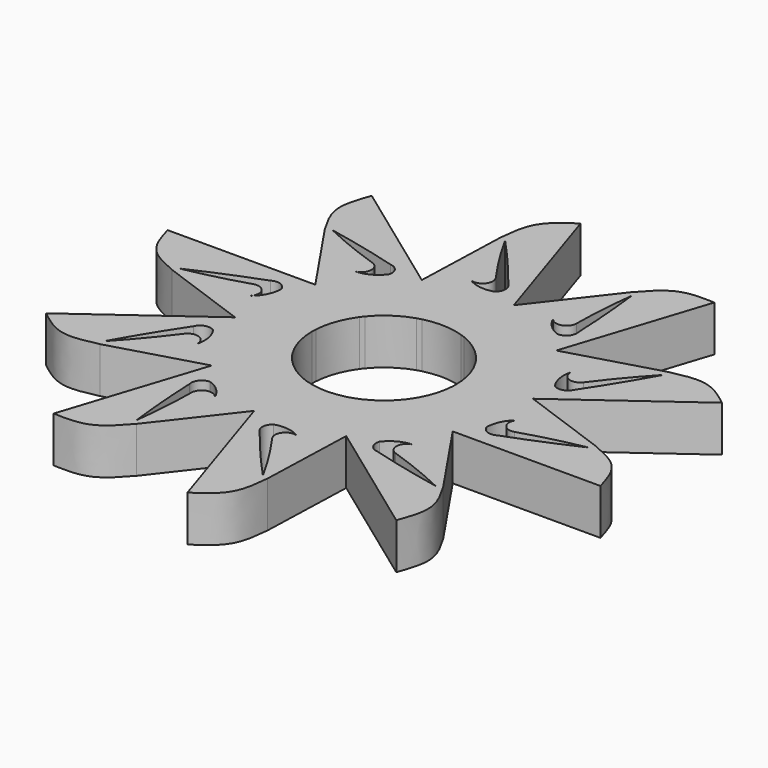
from build123d import *

# Parameters (mm, degrees)
F1_DEPTH      = 7
F3_DEPTH      = 80
F3_DEPTH_BACK = 25
F4_COUNT      = 10


# Not quite as in the source:
# - an extrude ends at something that could not be found from the text; its depth is read off the source's solid


with BuildPart() as f1:
    # F0 (on Top) → F1 (new body)
    with BuildSketch(Plane.XY):
        with BuildLine():
            ThreePointArc((9.2862347639, 5.8962567709), (10.5628732456, 3.0701317233), (11, 0))
            ThreePointArc((11, 0), (9.4389817008, -5.6485063912), (5.1989773724, -9.6938451752))
            Line((5.1989773724, -9.6938451752), (17.4936950276, -9.6938451752))
            ThreePointArc((17.4936950276, -9.6938451752), (19.3632887257, -5.0063010021), (20, 0))
            ThreePointArc((20, 0), (19.9371690623, 1.5840737934), (19.7490710217, 3.1581947026))
            Line((19.7490710217, 3.1581947026), (12.9913196682, 5.5989294212))
            ThreePointArc((12.9913196682, 5.5989294212), (12.1549883134, 5.8213640414), (11.2928291783, 5.8962567709))
            Line((11.2928291783, 5.8962567709), (9.2862347639, 5.8962567709))
        make_face()
        with BuildLine():
            ThreePointArc((5.1989773724, -9.6938451752), (-10.6404023576, 2.7895945347), (9.2862347639, 5.8962567709))
            Line((9.2862347639, 5.8962567709), (11.2928291783, 5.8962567709))
            ThreePointArc((11.2928291783, 5.8962567709), (12.1549883134, 5.8213640414), (12.9913196682, 5.5989294212))
            Line((12.9913196682, 5.5989294212), (19.7490710217, 3.1581947026))
            ThreePointArc((19.7490710217, 3.1581947026), (-19.6989755573, 3.4569295616), (17.4936950276, -9.6938451752))
            Line((17.4936950276, -9.6938451752), (5.1989773724, -9.6938451752))
        make_face()
        with BuildLine():
            ThreePointArc((20, 0), (19.3632887257, -5.0063010021), (17.4936950276, -9.6938451752))
            Line((17.4936950276, -9.6938451752), (40.8740527928, -9.6938451752))
            add(Edge.make_bspline(
                [(34.0516753495, -2.0075566135), (35.8141325987, -2.7740908853), (39.3168982789, -4.2975263847), (40.357193967, -7.9026709732), (40.8740527928, -9.6938451752)],
                knots=[0, 0, 0, 0, 0.5031616186, 1, 1, 1, 1], degree=3))
            Line((34.0516753495, -2.0075566135), (19.7490710217, 3.1581947026))
            ThreePointArc((19.7490710217, 3.1581947026), (19.9371690623, 1.5840737934), (20, 0))
        make_face()
    extrude(amount=F1_DEPTH)

    # F2 (on Top) → F3 (cut, two sides)
    with BuildSketch(Plane.XY) as f3_sk:
        with BuildLine():
            ThreePointArc((24.097783491, -5.1900828257), (22.3410218592, -4.5133442837), (22.484831512, -2.6362440549))
            ThreePointArc((22.484831512, -2.6362440549), (21.2063665687, -4.2559181051), (20.7374691963, -6.2653836794))
            ThreePointArc((20.7374691963, -6.2653836794), (21.7064439422, -7.2920152577), (23.1120903045, -7.1614673361))
            ThreePointArc((23.1120903045, -7.1614673361), (28.3759705314, -5.094612778), (33.5514694452, -2.8154607862))
            ThreePointArc((33.5514694452, -2.8154607862), (28.7888988276, -3.8605353205), (24.097783491, -5.1900828257))
        make_face()
    extrude(amount=-F3_DEPTH, mode=Mode.SUBTRACT)
    extrude(f3_sk.sketch, amount=F3_DEPTH_BACK, mode=Mode.SUBTRACT)

    # F4: F1 ×10 about axis
    f4_axis = Axis((0, 0, 7), (0, 0, 1))


with BuildPart() as f1_1:
    add(f1.part)
    for i in range(1, F4_COUNT):
        add(f1.part.rotate(f4_axis, i * 360 / F4_COUNT))


solid = f1_1.part
